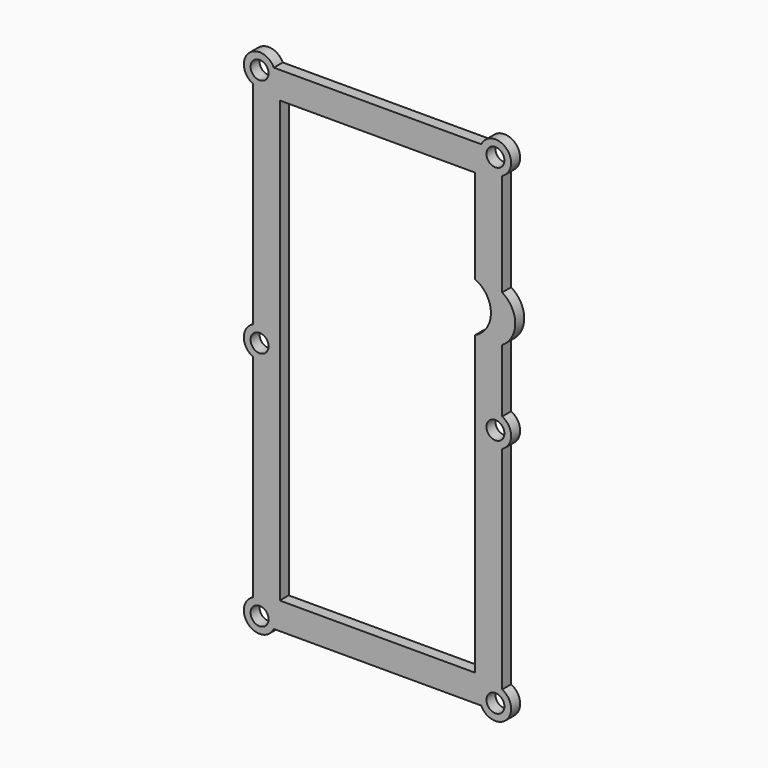
from build123d import *

# Parameters (mm, degrees)
F0_R     = 4
F1_DEPTH = 2.5
F3_DEPTH = 5


# Not quite as in the source:
# - a feature names something its author has since deleted; it is built from what else it names


with BuildPart() as f1:
    # F0 (on Front) → F1 (new body, symmetric)
    with BuildSketch(Plane.XZ):
        with BuildLine():
            Line((-58.4079127312, -18.8516896643), (-58.4079127312, -113.2025790236))
            ThreePointArc((-58.4079127312, -113.2025790236), (-60.3576601995, -124.4768818123), (-49.0833574108, -122.527134344))
            Line((-49.0833574108, -122.527134344), (43.2675319485, -122.527134344))
            ThreePointArc((43.2675319485, -122.527134344), (54.5418347371, -124.4768818123), (52.5920872688, -113.2025790236))
            Line((52.5920872688, -113.2025790236), (52.5920872688, -18.8516896643))
            ThreePointArc((52.5920872688, -18.8516896643), (56.5920872688, -12.527134344), (52.5920872688, -6.2025790236))
            Line((52.5920872688, -6.2025790236), (52.5920872688, 21.8966218341))
            ThreePointArc((52.5920872688, 21.8966218341), (58.408131243, 32.1608112925), (52.5920872688, 42.425000751))
            Line((52.5920872688, 42.425000751), (52.5920872688, 88.1483103357))
            ThreePointArc((52.5920872688, 88.1483103357), (54.5418347371, 99.4226131243), (43.2675319485, 97.472865656))
            Line((43.2675319485, 97.472865656), (-49.0833574108, 97.472865656))
            ThreePointArc((-49.0833574108, 97.472865656), (-60.3576601995, 99.4226131243), (-58.4079127312, 88.1483103357))
            Line((-58.4079127312, 88.1483103357), (-58.4079127312, -6.2025790236))
            ThreePointArc((-58.4079127312, -6.2025790236), (-62.4079127312, -12.527134344), (-58.4079127312, -18.8516896643))
        make_face()
        with Locations((-55.4079127312, -119.527134344)):
            Circle(F0_R, mode=Mode.SUBTRACT)
        with Locations((49.5920872688, -119.527134344)):
            Circle(F0_R, mode=Mode.SUBTRACT)
        with Locations((-55.4079127312, -12.527134344)):
            Circle(F0_R, mode=Mode.SUBTRACT)
        with Locations((-55.4079127312, 94.472865656)):
            Circle(F0_R, mode=Mode.SUBTRACT)
        with Locations((49.5920872688, -12.527134344)):
            Circle(F0_R, mode=Mode.SUBTRACT)
        with Locations((49.5920872688, 94.472865656)):
            Circle(F0_R, mode=Mode.SUBTRACT)
    extrude(amount=F1_DEPTH, both=True)

    # F2 (on Front) → F3 (cut, symmetric)
    with BuildSketch(Plane.XZ):
        with BuildLine():
            Line((40.5920872688, 85.472865656), (-46.4079127312, 85.472865656))
            Line((-46.4079127312, 85.472865656), (-46.4079127312, -110.527134344))
            Line((-46.4079127312, -110.527134344), (40.5920872688, -110.527134344))
            Line((40.5920872688, -110.527134344), (40.5920872688, 21.8337872246))
            ThreePointArc((40.5920872688, 21.8337872246), (47.5920872688, 32.7424993392), (40.5920872688, 43.6512114539))
            Line((40.5920872688, 43.6512114539), (40.5920872688, 85.472865656))
        make_face()
    extrude(amount=F3_DEPTH, both=True, mode=Mode.SUBTRACT)


solid = f1.part
